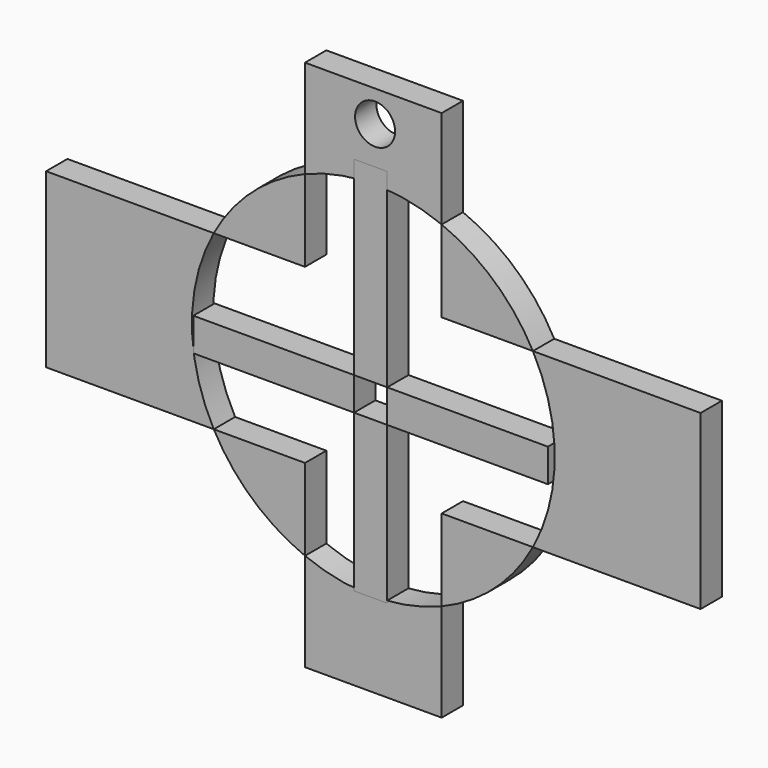
from build123d import *

# Parameters (mm, degrees)
F1_DEPTH = 25.4
F2_W     = 31.6208600998
F2_H     = 149.5748460293
F3_DEPTH = 25.4
F2_H_2   = 181.1054646969
F2_W_2   = 153.152346611
F2_H_3   = 31.5306186676
F5_D     = 38.1


with BuildPart() as f1:
    # F0 (on Front) → F1 (new body)
    with BuildSketch(Plane.XZ):
        with BuildLine():
            Line((818.0339336395, 288.8030409813), (818.0339336395, 382.2634366477))
            ThreePointArc((818.0339336395, 382.2634366477), (752.908706665, 369.5307429552), (687.7834796906, 382.2634366477))
            Line((687.7834796906, 382.2634366477), (687.7834796906, 288.8030409813))
            Line((687.7834796906, 288.8030409813), (818.0339336395, 288.8030409813))
        make_face()
    extrude(amount=F1_DEPTH)


with BuildPart() as f1b:
    # F0 (on Front) → F1, piece 2 (new body)
    with BuildSketch(Plane.XZ):
        with BuildLine():
            ThreePointArc((600.8124266323, 460.185110569), (579.9909885645, 542.4484610558), (600.8124266323, 624.7118115425))
            Line((600.8124266323, 624.7118115425), (440.9933388233, 624.7118115425))
            Line((440.9933388233, 624.7118115425), (440.9933388233, 460.185110569))
            Line((440.9933388233, 460.185110569), (600.8124266323, 460.185110569))
        make_face()
    extrude(amount=F1_DEPTH)


with BuildPart() as f1c:
    # F0 (on Front) → F1, piece 3 (new body)
    with BuildSketch(Plane.XZ):
        with BuildLine():
            ThreePointArc((600.8124266323, 460.185110569), (637.5213477678, 413.6606718838), (687.7834796906, 382.2634366477))
            Line((687.7834796906, 382.2634366477), (687.7834796906, 460.185110569))
            Line((687.7834796906, 460.185110569), (600.8124266323, 460.185110569))
        make_face()
    extrude(amount=F1_DEPTH)


with BuildPart() as f1d:
    # F0 (on Front) → F1, piece 4 (new body)
    with BuildSketch(Plane.XZ):
        with BuildLine():
            ThreePointArc((905.0049866977, 624.7118115425), (920.5402653107, 584.8771987123), (925.8264247656, 542.4484610558))
            ThreePointArc((925.8264247656, 542.4484610558), (920.5402653107, 500.0197233992), (905.0049866977, 460.185110569))
            Line((905.0049866977, 460.185110569), (1064.8240745068, 460.185110569))
            Line((1064.8240745068, 460.185110569), (1064.8240745068, 624.7118115425))
            Line((1064.8240745068, 624.7118115425), (905.0049866977, 624.7118115425))
        make_face()
    extrude(amount=F1_DEPTH)


with BuildPart() as f1e:
    # F0 (on Front) → F1, piece 5 (new body)
    with BuildSketch(Plane.XZ):
        with BuildLine():
            ThreePointArc((818.0339336395, 382.2634366477), (868.2960655623, 413.6606718838), (905.0049866977, 460.185110569))
            Line((905.0049866977, 460.185110569), (818.0339336395, 460.185110569))
            Line((818.0339336395, 460.185110569), (818.0339336395, 382.2634366477))
        make_face()
    extrude(amount=F1_DEPTH)


with BuildPart() as f1f:
    # F0 (on Front) → F1, piece 6 (new body)
    with BuildSketch(Plane.XZ):
        with BuildLine():
            Line((687.7834796906, 624.7118115425), (687.7834796906, 702.6334854638))
            ThreePointArc((687.7834796906, 702.6334854638), (637.5213477678, 671.2362502277), (600.8124266323, 624.7118115425))
            Line((600.8124266323, 624.7118115425), (687.7834796906, 624.7118115425))
        make_face()
    extrude(amount=F1_DEPTH)


with BuildPart() as f1g:
    # F0 (on Front) → F1, piece 7 (new body)
    with BuildSketch(Plane.XZ):
        with BuildLine():
            ThreePointArc((687.7834796906, 702.6334854638), (752.908706665, 715.3661791563), (818.0339336395, 702.6334854638))
            Line((818.0339336395, 702.6334854638), (818.0339336395, 796.0938811302))
            Line((818.0339336395, 796.0938811302), (687.7834796906, 796.0938811302))
            Line((687.7834796906, 796.0938811302), (687.7834796906, 702.6334854638))
        make_face()
    extrude(amount=F1_DEPTH)

    # F5 (through all)
    with Locations(Plane(origin=(0, 0, 0), x_dir=(1, 0, 0), z_dir=(0, 1, 0))):
        with Locations((754.5690536499, -766.2491202354)):
            Hole(F5_D / 2)


with BuildPart() as f1h:
    # F0 (on Front) → F1, piece 8 (new body)
    with BuildSketch(Plane.XZ):
        with BuildLine():
            Line((818.0339336395, 624.7118115425), (905.0049866977, 624.7118115425))
            ThreePointArc((905.0049866977, 624.7118115425), (868.2960655623, 671.2362502277), (818.0339336395, 702.6334854638))
            Line((818.0339336395, 702.6334854638), (818.0339336395, 624.7118115425))
        make_face()
    extrude(amount=F1_DEPTH)


with BuildPart() as f3:
    # F2 (on Front) → F3 (new body)
    with BuildSketch(Plane.XZ):
        with Locations((750.3167390823, 442.8054243326)):
            Rectangle(F2_W, F2_H)
    extrude(amount=F3_DEPTH)


with BuildPart() as f3b:
    # F2 (on Front) → F3, piece 2 (new body)
    with BuildSketch(Plane.XZ):
        with Locations((750.3167390823, 639.6761983633)):
            Rectangle(F2_W, F2_H_2)
    extrude(amount=F3_DEPTH)


with BuildPart() as f3c:
    # F2 (on Front) → F3, piece 3 (new body)
    with BuildSketch(Plane.XZ):
        with Locations((842.7033424377, 533.3581566811)):
            Rectangle(F2_W_2, F2_H_3)
    extrude(amount=F3_DEPTH)


with BuildPart() as f3d:
    # F2 (on Front) → F3, piece 4 (new body)
    with BuildSketch(Plane.XZ):
        with Locations((657.9301357269, 533.3581566811)):
            Rectangle(F2_W_2, F2_H_3)
    extrude(amount=F3_DEPTH)


solid = Compound([f1.part, f1b.part, f1c.part, f1d.part, f1e.part, f1f.part, f1g.part, f1h.part, f3.part, f3b.part, f3c.part, f3d.part])
